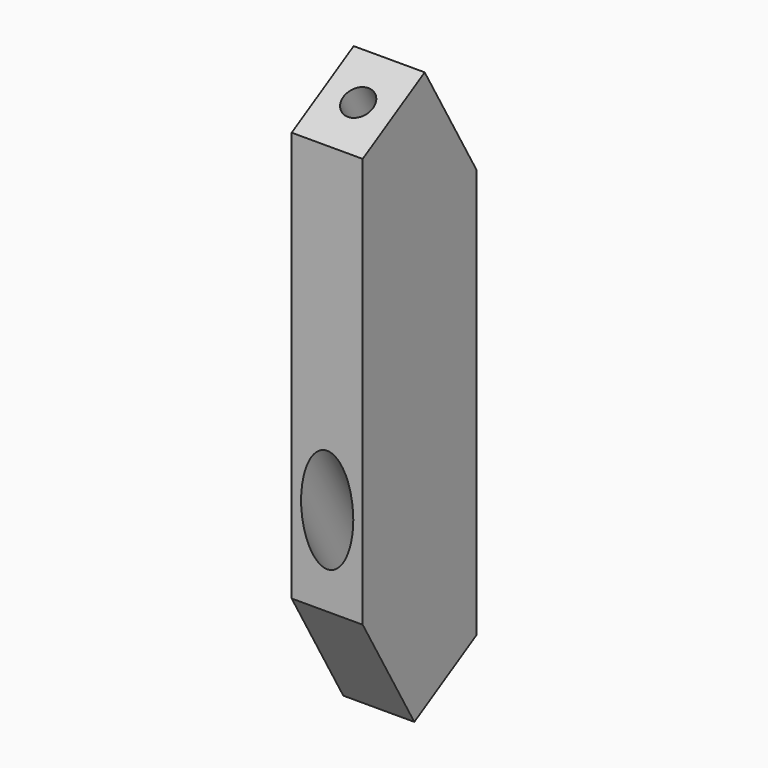
from build123d import *

# Parameters (mm, degrees)
F1_DEPTH = 4.7625
F2_R     = 2
F3_DEPTH = 50
F4_R     = 3.5
F4_R_2   = 2
F5_DEPTH = 40
F6_R     = 2
F7_DEPTH = 15.1971524227
F8_R     = 2
F9_DEPTH = 70.1490577065


# Not quite as in the source:
# - a length typed as a fraction of an inch, garbled in the dataset ("3 / 203.2 mm" for 3/8 in), is restored


with BuildPart() as f1:
    # F0 (on Right) → F1 (new body, symmetric)
    with BuildSketch(Plane.YZ):
        Polygon((0.8673048454, 75.500738686), (-9.525, 69.500738686), (-9.525, 14.4948291982), (-0.8673048454, -0.500738686), (9.525, 5.499261314), (9.525, 60.5051708018), align=None)
    extrude(amount=F1_DEPTH, both=True)

    # F2 (on face) → F3 (join)
    with BuildSketch(Plane(origin=(0, 0, 0), x_dir=(1, 0, 0), z_dir=(0, 0.5, -0.8660254038))):
        with Locations((0, -4.9985226281)):
            Circle(F2_R)
    extrude(amount=-F3_DEPTH)

    # F4 (on face) → F5 (cut)
    with BuildSketch(Plane(origin=(0, -25, 43.3012701892), x_dir=(1, 0, 0), z_dir=(0, -0.5, 0.8660254038))):
        with Locations((0, 4.9985226281)):
            Circle(F4_R)
        with Locations((0, 4.9985226281)):
            Circle(F4_R_2, mode=Mode.SUBTRACT)
        with Locations((0, 4.9985226281)):
            Circle(F4_R_2)
    extrude(amount=-F5_DEPTH, mode=Mode.SUBTRACT)

    # F6 (on face) → F7 (cut, through all)
    with BuildSketch(Plane(origin=(0, -5, 8.6602540378), x_dir=(1, 0, 0), z_dir=(0, -0.5, 0.8660254038))):
        with Locations((0, 4.9985226281)):
            Circle(F6_R)
    extrude(amount=-F7_DEPTH, mode=Mode.SUBTRACT)

    # F8 (on face) → F9 (cut, through all)
    with BuildSketch(Plane(origin=(0, -32.4759526419, 56.25), x_dir=(1, 0, 0), z_dir=(0, -0.5, 0.8660254038))):
        with Locations((0, 32.5014773719)):
            Circle(F8_R)
    extrude(amount=-F9_DEPTH, mode=Mode.SUBTRACT)


solid = f1.part
